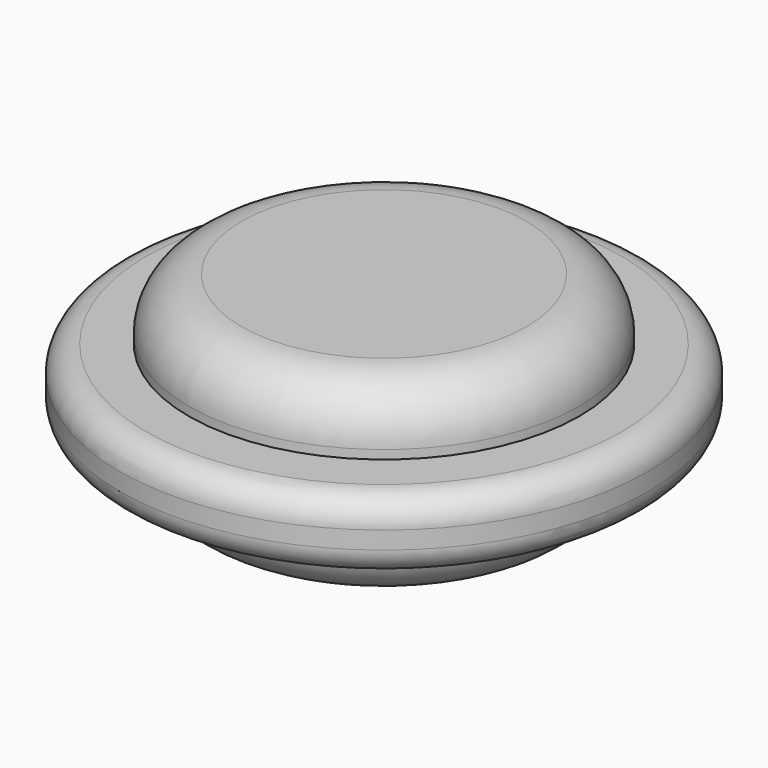
from build123d import *

# Parameters (mm, degrees)
F2_R     = 15
F2_R_2   = 11
F3_DEPTH = 2
F4_R     = 11.1
F5_DEPTH = 5.5
F6_R     = 3
F9_R     = 1.5


with BuildPart() as f3:
    # F2 (on Top) → F3 (new body, symmetric)
    with BuildSketch(Plane.XY):
        Circle(F2_R)
        Circle(F2_R_2, mode=Mode.SUBTRACT)
    extrude(amount=F3_DEPTH, both=True)


with BuildPart() as f5:
    # F4 (on Top) → F5 (new body, symmetric)
    with BuildSketch(Plane.XY):
        Circle(F4_R)
    extrude(amount=F5_DEPTH, both=True)

    # F6
    f6_edges = [f5.edges().sort_by_distance(p)[0] for p in [
        (-11.1, 0, 5.5),
        (-11.1, 0, -5.5),
    ]]
    fillet(f6_edges, radius=F6_R)


with BuildPart() as f7_1:
    # F7: copy of F3
    add(f3.part)


with BuildPart() as f5_1:
    add(f5.part)

    # F8: cut F7_1
    add(f7_1.part, mode=Mode.SUBTRACT)


with BuildPart() as f3_1:
    add(f3.part)

    # F9
    f9_edges = [f3_1.edges().sort_by_distance(p)[0] for p in [
        (-15, 0, -2),
        (15, 0, 0),
        (-15, 0, 2),
    ]]
    fillet(f9_edges, radius=F9_R)


solid = Compound([f5_1.part, f3_1.part])
